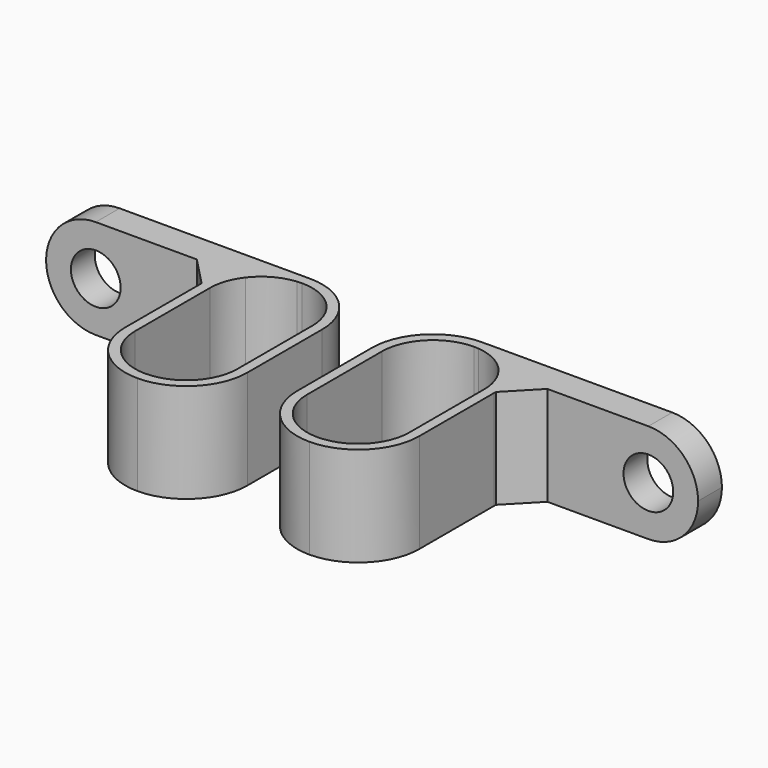
from build123d import *

# Parameters (mm, degrees)
F1_DEPTH      = 1
F2_DEPTH      = 10
F3_W          = 3
F3_H          = 10
F4_DEPTH      = 5.65
F4_DEPTH_BACK = 18
F6_DEPTH      = 9
F7_T1_DEPTH   = 10
F8_R          = 4.99999
F9_R          = 2.5
F10_DEPTH     = 25


# Not quite as in the source:
# - a fillet or chamfer that OpenCascade refuses, or shapes differently, is made with other operations: its cross-section is extruded or revolved along the edge and cut away or added
# - a fillet or chamfer is up to 0.001 mm smaller than in the source, because OpenCascade refuses the exact size


with BuildPart() as f1:
    # F0 (on Top) → F1 (new body)
    with BuildSketch(Plane.XY):
        with BuildLine():
            ThreePointArc((5.15, 0), (1.5084000769, -1.5084000769), (0, -5.15))
            Line((0, -5.15), (0, -14.55))
            ThreePointArc((0, -14.55), (1.5084000769, -18.1915999231), (5.15, -19.7))
            ThreePointArc((5.15, -19.7), (8.7915999231, -18.1915999231), (10.3, -14.55))
            Line((10.3, -14.55), (10.3, -5.15))
            ThreePointArc((10.3, -5.15), (8.7915999231, -1.5084000769), (5.15, 0))
        make_face()
    extrude(amount=F1_DEPTH)

    # F0 (on Top) → F2 (join)
    with BuildSketch(Plane.XY):
        with BuildLine():
            Line((11.3, -14.55), (11.3, -5.15))
            ThreePointArc((11.3, -5.15), (9.4987067043, -0.8012932957), (5.15, 1))
            ThreePointArc((5.15, 1), (0.8012932957, -0.8012932957), (-1, -5.15))
            Line((-1, -5.15), (-1, -14.55))
            ThreePointArc((-1, -14.55), (0.8012932957, -18.8987067043), (5.15, -20.7))
            ThreePointArc((5.15, -20.7), (9.4987067043, -18.8987067043), (11.3, -14.55))
        make_face()
        with BuildLine():
            Line((0, -14.55), (0, -5.15))
            ThreePointArc((0, -5.15), (1.5084000769, -1.5084000769), (5.15, 0))
            ThreePointArc((5.15, 0), (8.7915999231, -1.5084000769), (10.3, -5.15))
            Line((10.3, -5.15), (10.3, -14.55))
            ThreePointArc((10.3, -14.55), (8.7915999231, -18.1915999231), (5.15, -19.7))
            ThreePointArc((5.15, -19.7), (1.5084000769, -18.1915999231), (0, -14.55))
        make_face(mode=Mode.SUBTRACT)
    extrude(amount=F2_DEPTH)

    # F3 (on face) → F4 (join, two sides)
    with BuildSketch(Plane.YZ.offset(11.3)) as f4_sk:
        with Locations((-0.5, 5)):
            Rectangle(F3_W, F3_H)
    extrude(amount=-F4_DEPTH)
    extrude(f4_sk.sketch, amount=F4_DEPTH_BACK)

    # F5 (on face) → F6 (cut)
    with BuildSketch(Plane.XY.offset(10)):
        with BuildLine():
            Line((0, -5.15), (10.3, -5.15))
            ThreePointArc((10.3, -5.15), (10.0236636759, -3.4856976313), (9.2243097575, -2))
            Line((9.2243097575, -2), (5.65, -2))
            Line((5.65, -2), (5.65, -0.0243293122))
            ThreePointArc((5.65, -0.0243293122), (1.6896893203, -1.3357176298), (0, -5.15))
        make_face()
        with BuildLine():
            Line((5.65, -2), (9.2243097575, -2))
            ThreePointArc((9.2243097575, -2), (7.6413643062, -0.6427165727), (5.65, -0.0243293122))
            Line((5.65, -0.0243293122), (5.65, -2))
        make_face()
    extrude(amount=-F6_DEPTH, mode=Mode.SUBTRACT)

    # F7: chamfer of 5 on 1 edges, made by hand

    # F7_s2 → F7_t1 (join)
    with BuildSketch(Plane.XY):
        with BuildLine():
            Line((11.1573778033, -5.0816365025), (14.2734161404, -1.8561594829))
            Line((14.2734161404, -1.8561594829), (14.2734161404, -1.7561594829))
            ThreePointArc((14.2734161404, -1.7561594829), (12.3527305995, -1.9), (10.4320450585, -1.9))
            Line((10.4320450585, -1.9), (10.346158147, -2.0512195122))
            ThreePointArc((10.346158147, -2.0512195122), (10.9681971249, -3.4913613364), (11.0574373498, -5.0850869742))
            Line((11.0574373498, -5.0850869742), (11.1573778033, -5.0816365025))
        make_face()
    extrude(amount=F7_T1_DEPTH)

    # F8 (radius 5 in the source; OpenCascade refuses exactly that, so slightly less here)
    f8_edges = [f1.edges().sort_by_distance(p)[0] for p in [
        (29.3, -0.5, 10),
        (29.3, -0.5, 0),
    ]]
    fillet(f8_edges, radius=F8_R)

    # F9 (on face) → F10 (cut)
    with BuildSketch(Plane.XZ.offset(2)):
        with Locations((24.3, 5)):
            Circle(F9_R)
    extrude(amount=-F10_DEPTH, mode=Mode.SUBTRACT)


with BuildPart() as f11_1:
    # F11: instance of F1
    add(f1.part.mirror(Plane(origin=(-1, -9.85, 5), x_dir=(0, -1, 0), z_dir=(-1, 0, 0))))


with BuildPart() as f11_1_1:
    # F12: moved
    add(f11_1.part.moved(Location((-5, 0, 0))))


solid = Compound([f1.part, f11_1_1.part])
